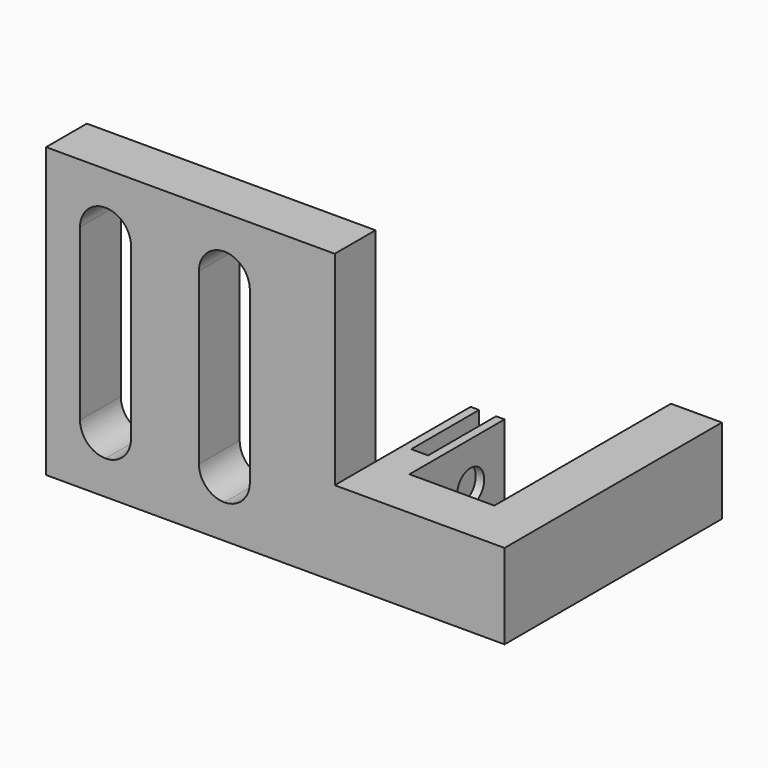
from build123d import *

# Parameters (mm, degrees)
F0_W      = 17
F0_H      = 17
F0_W_2    = 3
F0_H_2    = 13
F1_DEPTH  = 3
F2_W      = 3
F2_H      = 5
F3_DEPTH  = 10
F4_W      = 3
F4_H      = 5
F5_DEPTH  = 13
F6_W      = 2
F6_H      = 5
F7_DEPTH  = 7
F8_W      = 1
F8_H      = 5
F9_DEPTH  = 5
F10_R     = 1
F11_DEPTH = 3
F12_R     = 1.49999


# Not quite as in the source:
# - a fillet or chamfer is up to 0.001 mm smaller than in the source, because OpenCascade refuses the exact size


with BuildPart() as f1:
    # F0 (on Front) → F1 (new body)
    with BuildSketch(Plane.XZ):
        Rectangle(F0_W, F0_H)
        with Locations((-5, 0)):
            Rectangle(F0_W_2, F0_H_2, mode=Mode.SUBTRACT)
        with Locations((2, 0)):
            Rectangle(F0_W_2, F0_H_2, mode=Mode.SUBTRACT)
    extrude(amount=F1_DEPTH)

    # F2 (on face) → F3 (join)
    with BuildSketch(Plane.YZ.offset(8.5)):
        with Locations((-1.5, -6)):
            Rectangle(F2_W, F2_H)
    extrude(amount=F3_DEPTH)

    # F4 (on face) → F5 (join)
    with BuildSketch(Plane(origin=(0, 0, 0), x_dir=(-1, 0, 0), z_dir=(0, 1, 0))):
        with Locations((-17, -6)):
            Rectangle(F4_W, F4_H)
    extrude(amount=F5_DEPTH)

    # F6 (on face) → F7 (join)
    with BuildSketch(Plane(origin=(0, 0, 0), x_dir=(-1, 0, 0), z_dir=(0, 1, 0))):
        with Locations((-9.5, -6)):
            Rectangle(F6_W, F6_H)
    extrude(amount=F7_DEPTH)

    # F8 (on face) → F9 (cut)
    with BuildSketch(Plane(origin=(0, 7, 0), x_dir=(-1, 0, 0), z_dir=(0, 1, 0))):
        with Locations((-9.5, -6)):
            Rectangle(F8_W, F8_H)
    extrude(amount=-F9_DEPTH, mode=Mode.SUBTRACT)

    # F10 (on face) → F11 (cut)
    with BuildSketch(Plane(origin=(8.5, 0, 0), x_dir=(0, -1, 0), z_dir=(-1, 0, 0))):
        with Locations((-4.5, -6)):
            Circle(F10_R)
    extrude(amount=-F11_DEPTH, mode=Mode.SUBTRACT)

    # F12 (radius 1.5 in the source; OpenCascade refuses exactly that, so slightly less here)
    f12_edges = [f1.edges().sort_by_distance(p)[0] for p in [
        (-6.5, -1.5, 6.5),
        (0.5, -1.5, 6.5),
        (3.5, -1.5, 6.5),
        (-3.5, -1.5, 6.5),
        (-3.5, -1.5, -6.5),
        (3.5, -1.5, -6.5),
        (0.5, -1.5, -6.5),
        (-6.5, -1.5, -6.5),
    ]]
    fillet(f12_edges, radius=F12_R)


solid = f1.part
